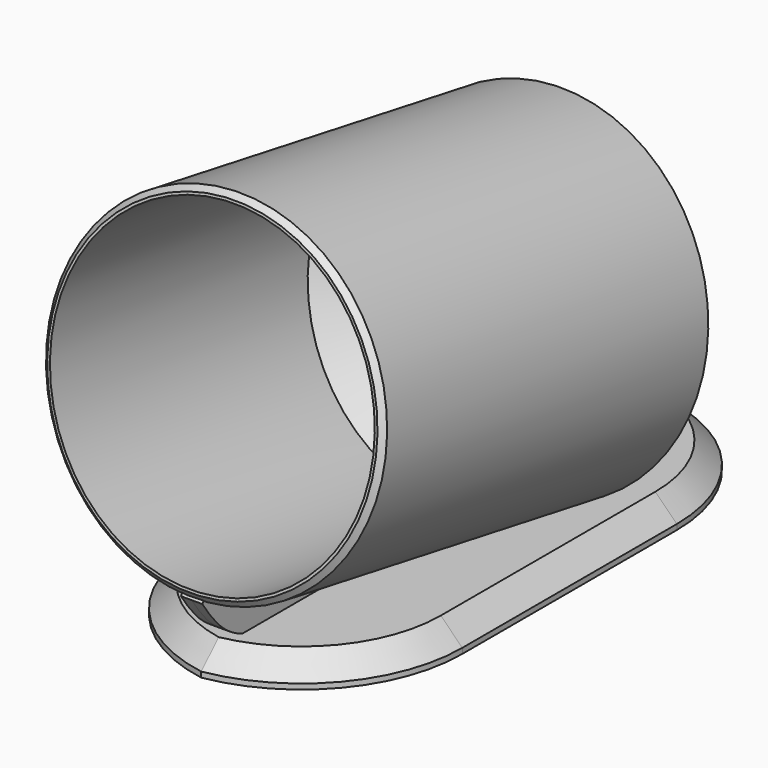
from build123d import *

# Parameters (mm, degrees)
F0_W          = 110
F0_H          = 5
F1_DEPTH      = 25
F3_R          = 31.5
F4_DEPTH      = 76
F4_DEPTH_BACK = 4
F5_D          = 60
F5_DEPTH      = 57
F5_TIP        = 18.0258185708
F5_2_D        = 60
F5_2_DEPTH    = 57
F5_2_TIP      = 18.0258185708
F6_D          = 60
F6_DEPTH      = 45
F6_TIP        = 18.0258185708
F8_D          = 8
F8_DEPTH      = 47
F8_TIP        = 2.4034424761
F8_2_D        = 8
F8_2_DEPTH    = 47
F8_2_TIP      = 2.4034424761
F10_DEPTH     = 2
F11_T1_DEPTH  = 155
F12_SIZE      = 3
F13_SIZE      = 1
F14_SIZE      = 4
F15_D         = 8
F15_DEPTH     = 47
F15_TIP       = 2.4034424761
F15_2_D       = 8
F15_2_DEPTH   = 47
F15_2_TIP     = 2.4034424761
F16_T1_DEPTH  = 4.2916195716
F16_T3_DEPTH  = 4.2916195716


# Not quite as in the source:
# - a fillet or chamfer that OpenCascade refuses, or shapes differently, is made with other operations: its cross-section is extruded or revolved along the edge and cut away or added


with BuildPart() as f1:
    # F0 (on Right) → F1 (new body, symmetric)
    with BuildSketch(Plane.YZ):
        Rectangle(F0_W, F0_H)
    extrude(amount=F1_DEPTH, both=True)

    # F5 (one way)
    with BuildSketch(Plane(origin=(0, -53.7690722508, 9.4809381655), x_dir=(1, 0, 0), z_dir=(0, -0.984807753, 0.1736481777))):
        with Locations((0, 32.9113696108)):
            Circle(F5_D / 2)
    extrude(amount=-F5_DEPTH, mode=Mode.SUBTRACT)
    with Locations(Plane(origin=(0, -53.7690722508, 9.4809381655), x_dir=(1, 0, 0), z_dir=(0, -0.984807753, 0.1736481777))):
        with Locations((0, 32.9113696108)):
            with Locations((0, 0, -(F5_DEPTH + F5_TIP / 2))):  # 118° drill point
                Cone(0, F5_D / 2, F5_TIP, mode=Mode.SUBTRACT)

    # F8 (one way)
    with BuildSketch(Plane.XY):
        with Locations((0, 13)):
            Circle(F8_D / 2)
    extrude(amount=-F8_DEPTH, mode=Mode.SUBTRACT)
    with Locations(Plane.XY):
        with Locations((0, 13)):
            with Locations((0, 0, -(F8_DEPTH + F8_TIP / 2))):  # 118° drill point
                Cone(0, F8_D / 2, F8_TIP, mode=Mode.SUBTRACT)

    # F11: fillet of radius 30 on 4 edges, made by hand

    # F11_s2 → F11_t1 (cut)
    with BuildSketch(Plane.XY.offset(-77.5)):
        with BuildLine():
            ThreePointArc((-25, -25), (-16.2132034356, -46.2132034356), (5, -55))
            Line((5, -55), (-25, -55))
            Line((-25, -55), (-25, -25))
        make_face()
        with BuildLine():
            ThreePointArc((-5, -55), (16.2132034356, -46.2132034356), (25, -25))
            Line((25, -25), (25, -55))
            Line((25, -55), (-5, -55))
        make_face()
        with BuildLine():
            ThreePointArc((-25, 25), (-16.2132034356, 46.2132034356), (5, 55))
            Line((5, 55), (-25, 55))
            Line((-25, 55), (-25, 25))
        make_face()
        with BuildLine():
            ThreePointArc((-5, 55), (16.2132034356, 46.2132034356), (25, 25))
            Line((25, 25), (25, 55))
            Line((25, 55), (-5, 55))
        make_face()
    extrude(amount=F11_T1_DEPTH, mode=Mode.SUBTRACT)

    # F14
    f14_edges = [f1.edges().sort_by_distance(p)[0] for p in [
        (17.912878, -44.364917, 2.5),
        (25, 0, 2.5),
        (17.912878, 44.364917, 2.5),
        (-17.912878, 44.364917, 2.5),
        (-25, 0, 2.5),
        (-17.912878, -44.364917, 2.5),
    ]]
    chamfer(f14_edges, length=F14_SIZE)

    # F15
    with Locations(Plane(origin=(0, 0, 0), x_dir=(1, 0, 0), z_dir=(0, 0, -1))):
        with Locations((0, -13)):
            Hole(F15_D / 2, depth=F15_DEPTH)
            with Locations((0, 0, -(F15_DEPTH + F15_TIP / 2))):  # 118° drill point
                Cone(0, F15_D / 2, F15_TIP, mode=Mode.SUBTRACT)


with BuildPart() as f4:
    # F3 (on face) → F4 (new body, two sides)
    with BuildSketch(Plane(origin=(0, -53.7690722508, 9.4809381655), x_dir=(1, 0, 0), z_dir=(0, -0.984807753, 0.1736481777))) as f4_sk:
        with Locations((0, 32.9113696108)):
            Circle(F3_R)
    extrude(amount=-F4_DEPTH)
    extrude(f4_sk.sketch, amount=F4_DEPTH_BACK)

    # F5#2 (one way)
    with BuildSketch(Plane(origin=(0, -53.7690722508, 9.4809381655), x_dir=(1, 0, 0), z_dir=(0, -0.984807753, 0.1736481777))):
        with Locations((0, 32.9113696108)):
            Circle(F5_2_D / 2)
    extrude(amount=-F5_2_DEPTH, mode=Mode.SUBTRACT)
    with Locations(Plane(origin=(0, -53.7690722508, 9.4809381655), x_dir=(1, 0, 0), z_dir=(0, -0.984807753, 0.1736481777))):
        with Locations((0, 32.9113696108)):
            with Locations((0, 0, -(F5_2_DEPTH + F5_2_TIP / 2))):  # 118° drill point
                Cone(0, F5_2_D / 2, F5_2_TIP, mode=Mode.SUBTRACT)

    # F6 (one way)
    with BuildSketch(Plane(origin=(0, -53.7690722508, 9.4809381655), x_dir=(1, 0, 0), z_dir=(0, 0.984807753, -0.1736481777))):
        with Locations((0, -32.9113696108)):
            Circle(F6_D / 2)
    extrude(amount=-F6_DEPTH, mode=Mode.SUBTRACT)
    with Locations(Plane(origin=(0, -53.7690722508, 9.4809381655), x_dir=(1, 0, 0), z_dir=(0, 0.984807753, -0.1736481777))):
        with Locations((0, -32.9113696108)):
            with Locations((0, 0, -(F6_DEPTH + F6_TIP / 2))):  # 118° drill point
                Cone(0, F6_D / 2, F6_TIP, mode=Mode.SUBTRACT)

    # F8#2 (one way)
    with BuildSketch(Plane.XY):
        with Locations((0, 13)):
            Circle(F8_2_D / 2)
    extrude(amount=-F8_2_DEPTH, mode=Mode.SUBTRACT)
    with Locations(Plane.XY):
        with Locations((0, 13)):
            with Locations((0, 0, -(F8_2_DEPTH + F8_2_TIP / 2))):  # 118° drill point
                Cone(0, F8_2_D / 2, F8_2_TIP, mode=Mode.SUBTRACT)

    # F12
    f12_edges = [f4.edges().sort_by_distance(p)[0] for p in [
        (-31.5, 26.791316, 28.695049),
    ]]
    chamfer(f12_edges, length=F12_SIZE)

    # F13
    f13_edges = [f4.edges().sort_by_distance(p)[0] for p in [
        (-31.5, -51.993304, 42.586903),
    ]]
    chamfer(f13_edges, length=F13_SIZE)

    # F15#2
    with Locations(Plane(origin=(0, 0, 0), x_dir=(1, 0, 0), z_dir=(0, 0, -1))):
        with Locations((0, -13)):
            Hole(F15_2_D / 2, depth=F15_2_DEPTH)
            with Locations((0, 0, -(F15_2_DEPTH + F15_2_TIP / 2))):  # 118° drill point
                Cone(0, F15_2_D / 2, F15_2_TIP, mode=Mode.SUBTRACT)


with BuildPart() as f10:
    # F9 (on Right) → F10 (new body, symmetric)
    with BuildSketch(Plane.YZ):
        with BuildLine():
            add(Edge.make_bspline(
                [(-26.9709937274, 0), (-35.2430958686, 0.1872683322), (-49.6820188119, 0.5141444964), (-55.0321186352, 8.4802371226), (-57.3171302676, 11.8825314566)],
                knots=[0, 0, 0, 0, 0.572902991, 1, 1, 1, 1], degree=3))
            Line((-26.9709937274, 0), (-5.1770457067, 0))
            Line((-5.1770457067, 0), (-5.1770457067, 2.8025961947))
            Line((-5.1770457067, 2.8025961947), (-57.3171302676, 11.8825314566))
        make_face()
    extrude(amount=F10_DEPTH, both=True)

    # F16: chamfer of 0.9 on 2 edges, made by hand

    # F16_s2 → F16_t1 (cut)
    with BuildSketch(Plane.YZ.offset(-4.2916195716)):
        with BuildLine():
            Line((-56.8331442384, 11.1040709469), (-56.4097543552, 11.7581442044))
            Line((-56.4097543552, 11.7581442044), (-56.4066662215, 11.7758773211))
            ThreePointArc((-56.4066662215, 11.7758773211), (-56.8631960445, 11.8217519791), (-57.3140421339, 11.9002645734))
            Line((-57.3140421339, 11.9002645734), (-57.3320729998, 11.8724957826))
            ThreePointArc((-57.3320729998, 11.8724957826), (-57.0766052058, 11.4923137573), (-56.8480585259, 11.0939930489))
            Line((-56.8480585259, 11.0939930489), (-56.8331442384, 11.1040709469))
        make_face()
    extrude(amount=F16_T1_DEPTH, mode=Mode.SUBTRACT)

    # F16_s4 → F16_t3 (cut)
    with BuildSketch(Plane.YZ):
        with BuildLine():
            Line((-56.8331442384, 11.1040709469), (-56.4097543552, 11.7581442044))
            Line((-56.4097543552, 11.7581442044), (-56.4066662215, 11.7758773211))
            ThreePointArc((-56.4066662215, 11.7758773211), (-56.8631960445, 11.8217519791), (-57.3140421339, 11.9002645734))
            Line((-57.3140421339, 11.9002645734), (-57.3320729998, 11.8724957826))
            ThreePointArc((-57.3320729998, 11.8724957826), (-57.0766052058, 11.4923137573), (-56.8480585259, 11.0939930489))
            Line((-56.8480585259, 11.0939930489), (-56.8331442384, 11.1040709469))
        make_face()
    extrude(amount=F16_T3_DEPTH, mode=Mode.SUBTRACT)


solid = Compound([f1.part, f4.part, f10.part])
